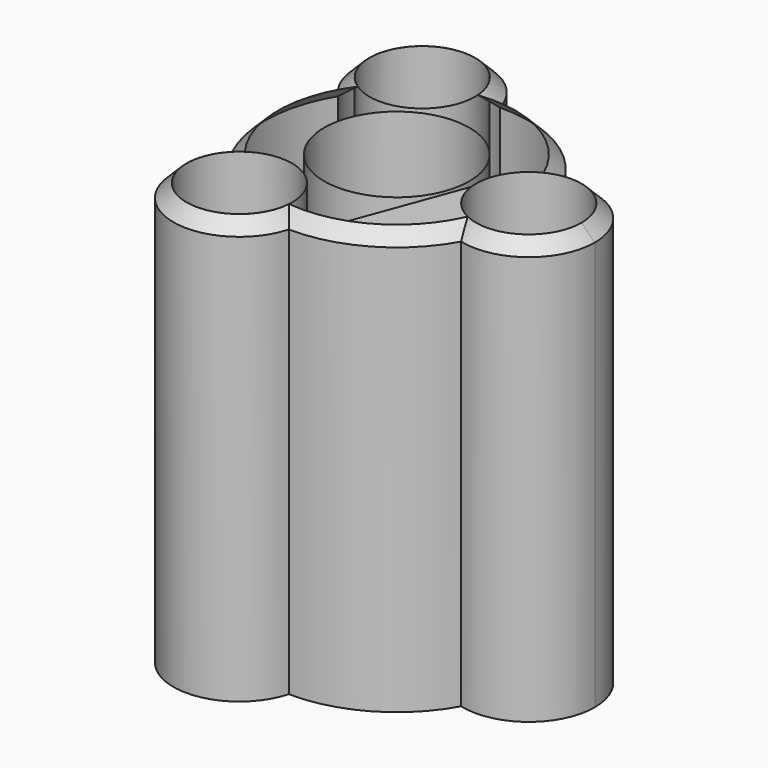
from build123d import *

# Parameters (mm, degrees)
F1_DEPTH = 160
F2_DEPTH = 160
F3_R     = 20
F3_R_2   = 27.5
F4_DEPTH = 50
F5_SIZE  = 4.99999


# Not quite as in the source:
# - a fillet or chamfer is up to 0.001 mm smaller than in the source, because OpenCascade refuses the exact size


with BuildPart() as f1:
    # F0 (on Top) → F1 (new body)
    with BuildSketch(Plane.XY):
        with BuildLine():
            ThreePointArc((43.75, 24.2061459138), (48.4122918276, 12.5), (50, 0))
            ThreePointArc((50, 0), (48.4122918276, -12.5), (43.75, -24.2061459138))
            ThreePointArc((43.75, -24.2061459138), (65.3093108924, -19.7642353761), (75, 0))
            ThreePointArc((75, 0), (65.3093108924, 19.7642353761), (43.75, 24.2061459138))
        make_face()
        with BuildLine():
            ThreePointArc((43.75, -24.2061459138), (48.4122918276, -12.5), (50, 0))
            ThreePointArc((50, 0), (48.4122918276, 12.5), (43.75, 24.2061459138))
            ThreePointArc((43.75, 24.2061459138), (25, 0), (43.75, -24.2061459138))
        make_face()
        with BuildLine():
            ThreePointArc((43.75, -24.2061459138), (25, 0), (43.75, 24.2061459138))
            ThreePointArc((43.75, 24.2061459138), (25, 43.3012701892), (-0.9118627109, 49.9916843725))
            ThreePointArc((-0.9118627109, 49.9916843725), (-0.2290146318, 46.6774046484), (0, 43.3012701892))
            ThreePointArc((0, 43.3012701892), (-15.5383255242, 20.1609003539), (-42.8381372891, 25.7855384587))
            ThreePointArc((-42.8381372891, 25.7855384587), (-50, 0), (-42.8381372891, -25.7855384587))
            ThreePointArc((-42.8381372891, -25.7855384587), (-15.5383255242, -20.1609003539), (0, -43.3012701892))
            ThreePointArc((0, -43.3012701892), (-0.2290146318, -46.6774046484), (-0.9118627109, -49.9916843725))
            ThreePointArc((-0.9118627109, -49.9916843725), (25, -43.3012701892), (43.75, -24.2061459138))
        make_face()
    extrude(amount=F1_DEPTH)

    # F0 (on Top) → F2 (join)
    with BuildSketch(Plane.XY):
        with BuildLine():
            ThreePointArc((-42.8381372891, 25.7855384587), (-25, 43.3012701892), (-0.9118627109, 49.9916843725))
            ThreePointArc((-0.9118627109, 49.9916843725), (-37.5, 64.9519052838), (-42.8381372891, 25.7855384587))
        make_face()
        with BuildLine():
            ThreePointArc((0, 43.3012701892), (-0.2290146318, 46.6774046484), (-0.9118627109, 49.9916843725))
            ThreePointArc((-0.9118627109, 49.9916843725), (-25, 43.3012701892), (-42.8381372891, 25.7855384587))
            ThreePointArc((-42.8381372891, 25.7855384587), (-15.5383255242, 20.1609003539), (0, 43.3012701892))
        make_face()
        with BuildLine():
            ThreePointArc((43.75, -24.2061459138), (25, 0), (43.75, 24.2061459138))
            ThreePointArc((43.75, 24.2061459138), (25, 43.3012701892), (-0.9118627109, 49.9916843725))
            ThreePointArc((-0.9118627109, 49.9916843725), (-0.2290146318, 46.6774046484), (0, 43.3012701892))
            ThreePointArc((0, 43.3012701892), (-15.5383255242, 20.1609003539), (-42.8381372891, 25.7855384587))
            ThreePointArc((-42.8381372891, 25.7855384587), (-50, 0), (-42.8381372891, -25.7855384587))
            ThreePointArc((-42.8381372891, -25.7855384587), (-15.5383255242, -20.1609003539), (0, -43.3012701892))
            ThreePointArc((0, -43.3012701892), (-0.2290146318, -46.6774046484), (-0.9118627109, -49.9916843725))
            ThreePointArc((-0.9118627109, -49.9916843725), (25, -43.3012701892), (43.75, -24.2061459138))
        make_face()
        with BuildLine():
            ThreePointArc((43.75, -24.2061459138), (48.4122918276, -12.5), (50, 0))
            ThreePointArc((50, 0), (48.4122918276, 12.5), (43.75, 24.2061459138))
            ThreePointArc((43.75, 24.2061459138), (25, 0), (43.75, -24.2061459138))
        make_face()
        with BuildLine():
            ThreePointArc((43.75, 24.2061459138), (48.4122918276, 12.5), (50, 0))
            ThreePointArc((50, 0), (48.4122918276, -12.5), (43.75, -24.2061459138))
            ThreePointArc((43.75, -24.2061459138), (65.3093108924, -19.7642353761), (75, 0))
            ThreePointArc((75, 0), (65.3093108924, 19.7642353761), (43.75, 24.2061459138))
        make_face()
        with BuildLine():
            ThreePointArc((-42.8381372891, -25.7855384587), (-25, -43.3012701892), (-0.9118627109, -49.9916843725))
            ThreePointArc((-0.9118627109, -49.9916843725), (-0.2290146318, -46.6774046484), (0, -43.3012701892))
            ThreePointArc((0, -43.3012701892), (-15.5383255242, -20.1609003539), (-42.8381372891, -25.7855384587))
        make_face()
        with BuildLine():
            ThreePointArc((-42.8381372891, -25.7855384587), (-37.5, -64.9519052838), (-0.9118627109, -49.9916843725))
            ThreePointArc((-0.9118627109, -49.9916843725), (-25, -43.3012701892), (-42.8381372891, -25.7855384587))
        make_face()
    extrude(amount=F2_DEPTH)

    # F3 (on face) → F4 (cut)
    with BuildSketch(Plane.XY.offset(160)):
        with Locations((-25, 43.3012701892)):
            Circle(F3_R)
        with Locations((-25, -43.3012701892)):
            Circle(F3_R)
        with Locations((50, 0)):
            Circle(F3_R)
        Circle(F3_R_2)
    extrude(amount=-F4_DEPTH, mode=Mode.SUBTRACT)

    # F5 (size 5 in the source; OpenCascade refuses exactly that, so slightly less here)
    f5_edges = [f1.edges().sort_by_distance(p)[0] for p in [
        (25, -43.30127, 160),
        (-37.5, -64.951905, 160),
        (-50, 0, 160),
        (-37.5, 64.951905, 160),
        (25, 43.30127, 160),
        (75, 0, 160),
    ]]
    chamfer(f5_edges, length=F5_SIZE)


solid = f1.part
